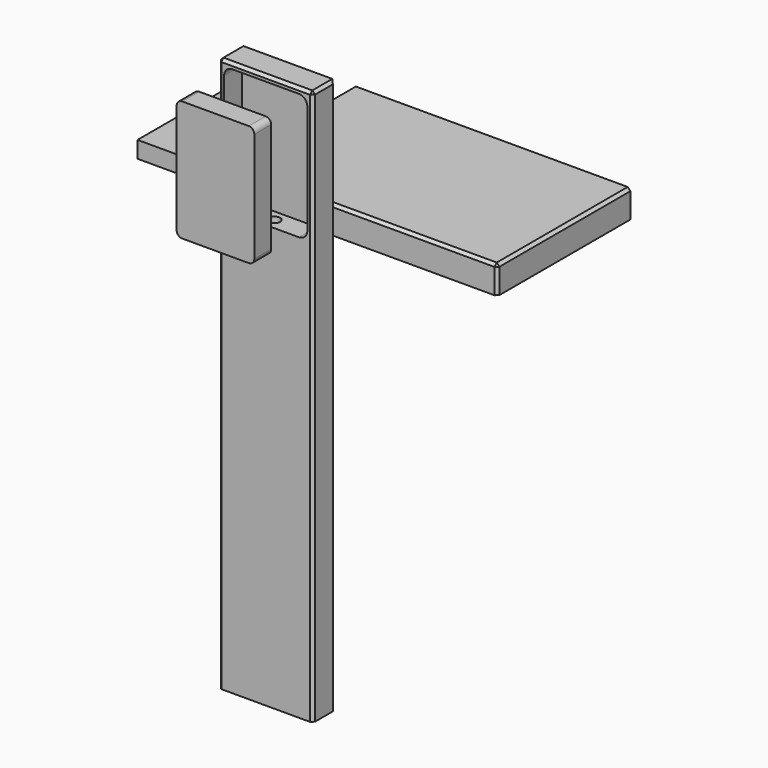
from build123d import *

# Parameters (mm, degrees)
F1_DEPTH  = 7.63
F2_R      = 1
F3_DEPTH  = 3.68
F4_W      = 8
F4_H      = 5.62
F5_DEPTH  = 0.82
F6_R      = 1.25
F7_DEPTH  = 1.67
F9_DEPTH  = 5.6
F10_W     = 21
F10_H     = 49.5
F11_DEPTH = 6
F12_W     = 34
F12_H     = 200
F13_DEPTH = 10
F16_DEPTH = 8
F17_R     = 2
F18_DEPTH = 152.5
F19_R     = 0.75
F20_DEPTH = 2
F21_SIZE  = 1
F22_W     = 100
F22_H     = 60
F23_DEPTH = 10
F24_SIZE  = 1
F26_DEPTH = 8


with BuildPart() as f1:
    # F0 (on Front) → F1 (new body)
    with BuildSketch(Plane.XZ):
        with BuildLine():
            Line((7.4422570039, 49.1264154027), (-16.5577429961, 49.1264154027))
            ThreePointArc((-16.5577429961, 49.1264154027), (-17.9719565585, 48.5406289651), (-18.5577429961, 47.1264154027))
            Line((-18.5577429961, 47.1264154027), (-18.5577429961, 7.6264154027))
            ThreePointArc((-18.5577429961, 7.6264154027), (-17.9719565585, 6.2122018403), (-16.5577429961, 5.6264154027))
            Line((-16.5577429961, 5.6264154027), (7.4422570039, 5.6264154027))
            ThreePointArc((7.4422570039, 5.6264154027), (8.8564705662, 6.2122018403), (9.4422570039, 7.6264154027))
            Line((9.4422570039, 7.6264154027), (9.4422570039, 47.1264154027))
            ThreePointArc((9.4422570039, 47.1264154027), (8.8564705662, 48.5406289651), (7.4422570039, 49.1264154027))
        make_face()
    extrude(amount=F1_DEPTH)


with BuildPart() as f3:
    # F2 (on Top) → F3 (new body)
    with BuildSketch(Plane.XY):
        with BuildLine():
            ThreePointArc((-28.4477795787, 7.5124184459), (-27.8619931411, 6.0982048835), (-26.4477795787, 5.5124184459))
            Line((-26.4477795787, 5.5124184459), (-12.6477795787, 5.5124184459))
            ThreePointArc((-12.6477795787, 5.5124184459), (-11.2335660163, 6.0982048835), (-10.6477795787, 7.5124184459))
            Line((-10.6477795787, 7.5124184459), (-10.6477795787, 40.8924184459))
            ThreePointArc((-10.6477795787, 40.8924184459), (-11.2335660163, 42.3066320083), (-12.6477795787, 42.8924184459))
            Line((-12.6477795787, 42.8924184459), (-26.4477795787, 42.8924184459))
            ThreePointArc((-26.4477795787, 42.8924184459), (-27.8619931411, 42.3066320083), (-28.4477795787, 40.8924184459))
            Line((-28.4477795787, 40.8924184459), (-28.4477795787, 7.5124184459))
        make_face()
        with Locations((-26.4477795787, 40.8924184459)):
            Circle(F2_R, mode=Mode.SUBTRACT)
        with Locations((-12.6477795787, 40.8924184459)):
            Circle(F2_R, mode=Mode.SUBTRACT)
    extrude(amount=F3_DEPTH)

    # F4 (on face) → F5 (join)
    with BuildSketch(Plane.XY.offset(3.68)):
        with Locations((-19.5477795787, 40.0824184459)):
            Rectangle(F4_W, F4_H)
    extrude(amount=F5_DEPTH)


with BuildPart() as f7:
    # F6 (on Top) → F7 (new body)
    with BuildSketch(Plane.XY):
        with BuildLine():
            Line((11.649762845, 10.926425495), (22.449762845, 10.926425495))
            ThreePointArc((22.449762845, 10.926425495), (23.8639764074, 11.5122119326), (24.449762845, 12.926425495))
            Line((24.449762845, 12.926425495), (24.449762845, 25.596425495))
            ThreePointArc((24.449762845, 25.596425495), (23.8639764074, 27.0106390574), (22.449762845, 27.596425495))
            Line((22.449762845, 27.596425495), (11.149762845, 27.596425495))
            ThreePointArc((11.149762845, 27.596425495), (9.7355492827, 27.0106390574), (9.149762845, 25.596425495))
            Line((9.149762845, 25.596425495), (9.149762845, 13.426425495))
            ThreePointArc((9.149762845, 13.426425495), (9.8819958921, 11.658658542), (11.649762845, 10.926425495))
        make_face()
        with Locations((22.449762845, 12.926425495)):
            Circle(F6_R, mode=Mode.SUBTRACT)
    extrude(amount=F7_DEPTH)

    # F8 (on face) → F9 (join)
    with BuildSketch(Plane.XY.offset(1.67)):
        with BuildLine():
            ThreePointArc((11.149762845, 10.9769357522), (11.39849044, 10.9390851125), (11.649762845, 10.926425495))
            Line((11.649762845, 10.926425495), (19.149762845, 10.926425495))
            Line((19.149762845, 10.926425495), (19.149762845, 16.926425495))
            Line((19.149762845, 16.926425495), (11.149762845, 16.926425495))
            Line((11.149762845, 16.926425495), (11.149762845, 10.9769357522))
        make_face()
    extrude(amount=F9_DEPTH)


with BuildPart() as f11:
    # F10 (on Top) → F11 (new body)
    with BuildSketch(Plane.XY):
        with Locations((-52.9828201979, 30.6568196436)):
            Rectangle(F10_W, F10_H)
    extrude(amount=F11_DEPTH)


with BuildPart() as f13:
    # F12 (on Front) → F13 (new body)
    with BuildSketch(Plane.XZ):
        with Locations((-4.5577429961, -47.8735845973)):
            Rectangle(F12_W, F12_H)
    extrude(amount=F13_DEPTH)

    # F15 (on face) → F16 (cut)
    with BuildSketch(Plane.XZ.offset(10)):
        with BuildLine():
            Line((7.4422570039, 50.1264154027), (-16.5577429961, 50.1264154027))
            ThreePointArc((-16.5577429961, 50.1264154027), (-18.6790633397, 49.2477357463), (-19.5577429961, 47.1264154027))
            Line((-19.5577429961, 47.1264154027), (-19.5577429961, 7.6264154027))
            ThreePointArc((-19.5577429961, 7.6264154027), (-18.6790633397, 5.5050950591), (-16.5577429961, 4.6264154027))
            Line((-16.5577429961, 4.6264154027), (7.4422570039, 4.6264154027))
            ThreePointArc((7.4422570039, 4.6264154027), (9.5635773474, 5.5050950591), (10.4422570039, 7.6264154027))
            Line((10.4422570039, 7.6264154027), (10.4422570039, 47.1264154027))
            ThreePointArc((10.4422570039, 47.1264154027), (9.5635773474, 49.2477357463), (7.4422570039, 50.1264154027))
        make_face()
    extrude(amount=-F16_DEPTH, mode=Mode.SUBTRACT)

    # F17 (on face) → F18 (cut, through all)
    with BuildSketch(Plane(origin=(0, 0, -147.8735845973), x_dir=(1, 0, 0), z_dir=(0, 0, -1))):
        with Locations((-4.5577429961, 6)):
            Circle(F17_R)
    extrude(amount=-F18_DEPTH, mode=Mode.SUBTRACT)

    # F19 (on face) → F20 (cut, through all)
    with BuildSketch(Plane.XZ.offset(2)):
        with Locations((-16.5577429961, 47.1264154027)):
            Circle(F19_R)
        with Locations((7.4422570039, 47.1264154027)):
            Circle(F19_R)
        with Locations((7.4422570039, 7.6264154027)):
            Circle(F19_R)
        with Locations((-16.5577429961, 7.6264154027)):
            Circle(F19_R)
    extrude(amount=-F20_DEPTH, mode=Mode.SUBTRACT)

    # F21
    f21_edges = [f13.edges().sort_by_distance(p)[0] for p in [
        (12.442257, -5, 52.126415),
        (-4.557743, -10, 52.126415),
        (12.442257, -10, -47.873585),
        (12.442257, 0, -47.873585),
        (-21.557743, -10, -47.873585),
        (-21.557743, -5, 52.126415),
    ]]
    chamfer(f21_edges, length=F21_SIZE)


with BuildPart() as f1_1:
    # F14: moved
    add(f1.part.moved(Location((0, -25, 0))))


with BuildPart() as f23:
    # F22 (on Top) → F23 (new body)
    with BuildSketch(Plane.XY):
        with Locations((17.9768048227, 33.69845354)):
            Rectangle(F22_W, F22_H)
    extrude(amount=F23_DEPTH)

    # F24
    f24_edges = [f23.edges().sort_by_distance(p)[0] for p in [
        (67.976805, 3.698454, 5),
        (67.976805, 33.698454, 10),
        (17.976805, 3.698454, 10),
        (-32.023195, 33.698454, 10),
        (-32.023195, 3.698454, 5),
    ]]
    chamfer(f24_edges, length=F24_SIZE)

    # F25 (on face) → F26 (cut)
    with BuildSketch(Plane(origin=(0, 0, 0), x_dir=(1, 0, 0), z_dir=(0, 0, -1))):
        with BuildLine():
            ThreePointArc((57.9768048227, -19.69845354), (56.2194455098, -15.4558128529), (51.9768048227, -13.69845354))
            Line((51.9768048227, -13.69845354), (-16.0231951773, -13.69845354))
            ThreePointArc((-16.0231951773, -13.69845354), (-20.2658358644, -15.4558128529), (-22.0231951773, -19.69845354))
            Line((-22.0231951773, -19.69845354), (-22.0231951773, -47.69845354))
            ThreePointArc((-22.0231951773, -47.69845354), (-20.2658358644, -51.9410942271), (-16.0231951773, -53.69845354))
            Line((-16.0231951773, -53.69845354), (31.9768048227, -53.69845354))
            Line((31.9768048227, -53.69845354), (31.9768048227, -63.69845354))
            Line((31.9768048227, -63.69845354), (51.9768048227, -63.69845354))
            Line((51.9768048227, -63.69845354), (51.9768048227, -53.69845354))
            ThreePointArc((51.9768048227, -53.69845354), (56.2194455098, -51.9410942271), (57.9768048227, -47.69845354))
            Line((57.9768048227, -47.69845354), (57.9768048227, -19.69845354))
        make_face()
    extrude(amount=-F26_DEPTH, mode=Mode.SUBTRACT)


solid = Compound([f3.part, f7.part, f11.part, f13.part, f1_1.part, f23.part])
